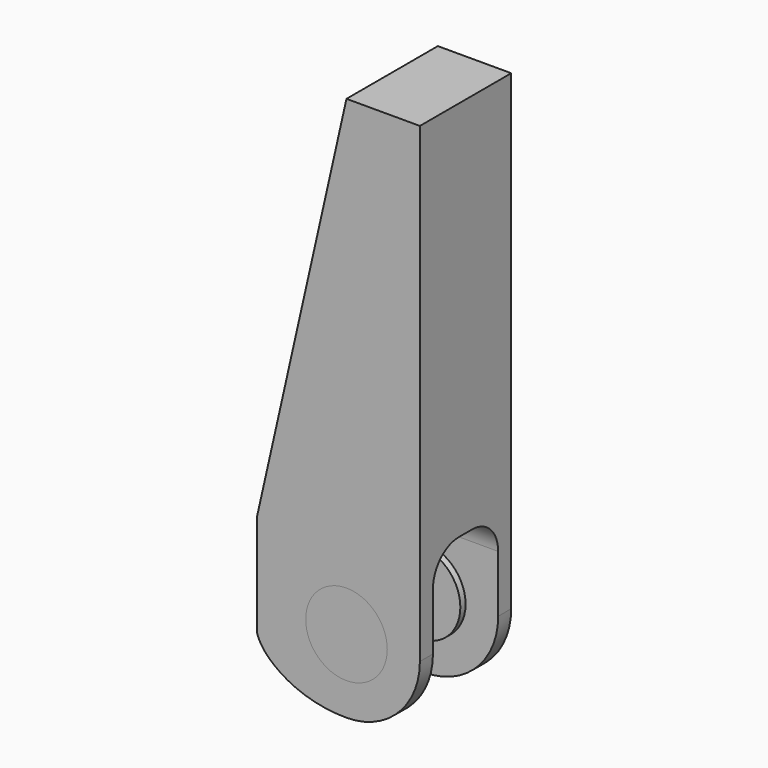
from build123d import *

# Parameters (mm, degrees)
F0_R      = 5
F1_DEPTH  = 14
F2_W      = 10
F2_H      = 9
F2_H_2    = 11
F3_DEPTH  = 25
F5_R      = 5
F6_DEPTH  = 14
F7_W      = 5
F7_H      = 8.4
F8_DEPTH  = 66.8020807441
F10_D     = 4.9784
F9_R      = 4
F11_DEPTH = 2
F12_R     = 4


with BuildPart() as f1:
    # F0 (on Front) → F1 (new body)
    with BuildSketch(Plane.XZ):
        with BuildLine():
            ThreePointArc((0, 0), (6.3639610307, 2.6360389693), (9, 9))
            Line((9, 9), (9, 66.8010806441))
            Line((9, 66.8010806441), (0, 66.8010806441))
            Line((0, 66.8010806441), (-11, 18))
            Line((-11, 18), (-11, 6))
            add(Edge.make_bspline(
                [(-11, 6), (-11, 4), (-7, 0), (0, 0)],
                knots=[0, 0, 0, 0, 12.5299640861, 12.5299640861, 12.5299640861, 12.5299640861], degree=3))
        make_face()
        with Locations((0, 9)):
            Circle(F0_R, mode=Mode.SUBTRACT)
    extrude(amount=F1_DEPTH)

    # F2 (on face) → F3 (cut)
    with BuildSketch(Plane.YZ.offset(9)):
        with Locations((-7, 4.5)):
            Rectangle(F2_W, F2_H)
        with Locations((-7, 14.5)):
            Rectangle(F2_W, F2_H_2)
    extrude(amount=-F3_DEPTH, mode=Mode.SUBTRACT)

    # F12
    f12_edges = [f1.edges().sort_by_distance(p)[0] for p in [
        (-0.774595, -12, 20),
        (-0.774595, -2, 20),
    ]]
    fillet(f12_edges, radius=F12_R)


with BuildPart() as f6:
    # F5 (on face) → F6 (new body, through all)
    with BuildSketch(Plane.XZ.offset(14)):
        with Locations((0, 9)):
            Circle(F5_R)
    extrude(amount=-F6_DEPTH)

    # F7 (on Top) → F8 (cut, through all)
    with BuildSketch(Plane.XY):
        with Locations((2.5, -7)):
            Rectangle(F7_W, F7_H)
    extrude(amount=F8_DEPTH, mode=Mode.SUBTRACT)

    # F10 (through all)
    with Locations(Plane.YZ):
        with Locations((-7, 9)):
            Hole(F10_D / 2)

    # F9 (on face) → F11 (cut)
    with BuildSketch(Plane.YZ):
        with Locations((-7, 9)):
            Circle(F9_R)
    extrude(amount=-F11_DEPTH, mode=Mode.SUBTRACT)


solid = Compound([f1.part, f6.part])
